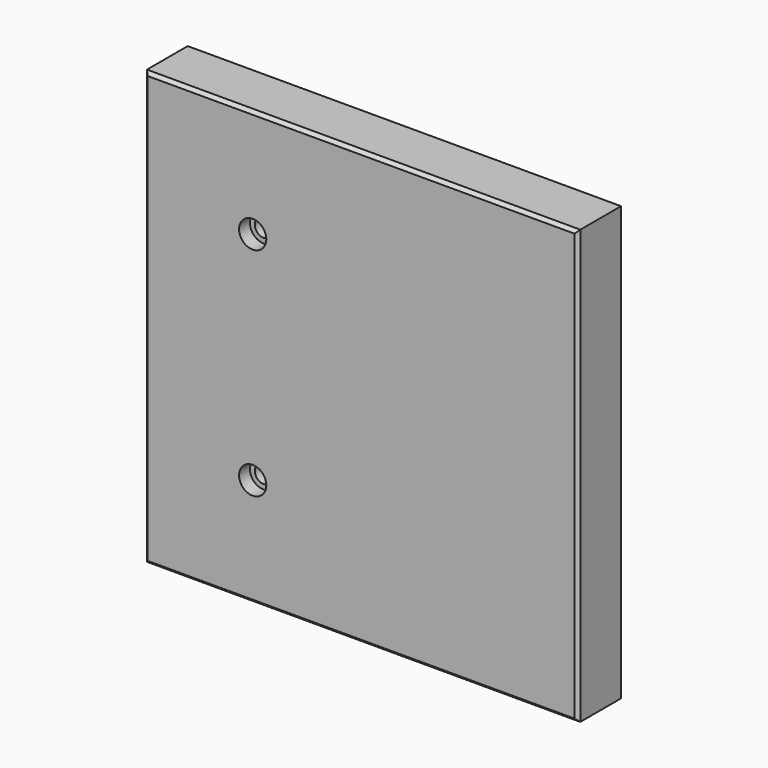
from build123d import *

# Parameters (mm, degrees)
F0_W     = 203.2
F0_H     = 203.2
F1_DEPTH = 12.7
F2_SIZE  = 1.524
F3_R     = 12.7
F4_DEPTH = 25.401
F5_R     = 12.7
F5_R_2   = 4.09575
F6_DEPTH = 12.7
F7_R     = 6.3754
F8_DEPTH = 6.35


# Not quite as in the source:
# - a pattern or mirror of a feature is missing from the dataset's text; its kind, count and spacing are read off the source's solid


with BuildPart() as f1:
    # F0 (on Front) → F1 (new body, symmetric)
    with BuildSketch(Plane.XZ):
        Rectangle(F0_W, F0_H)
    extrude(amount=F1_DEPTH, both=True)

    # F2
    f2_edges = [f1.edges().sort_by_distance(p)[0] for p in [
        (101.6, -12.7, 0),
        (0, -12.7, 101.6),
        (-101.6, -12.7, 0),
        (0, -12.7, -101.6),
    ]]
    chamfer(f2_edges, length=F2_SIZE)

    # F3 (on face) → F4 (cut, through all)
    with BuildSketch(Plane.XZ.offset(12.7)):
        with Locations((-50.8, -50.8)):
            Circle(F3_R)
    f4 = extrude(amount=-F4_DEPTH, mode=Mode.SUBTRACT)

    # F4_copies: F4 across plane
    add(f4.mirror(Plane.XY), mode=Mode.SUBTRACT)

    # F5 (on face) → F6 (join)
    with BuildSketch(Plane.XZ.offset(12.7)):
        with Locations((-50.8, 50.8)):
            Circle(F5_R)
        with Locations((-50.8, 50.8)):
            Circle(F5_R_2, mode=Mode.SUBTRACT)
        with Locations((-50.8, -50.8)):
            Circle(F5_R)
        with Locations((-50.8, -50.8)):
            Circle(F5_R_2, mode=Mode.SUBTRACT)
    extrude(amount=-F6_DEPTH)

    # F7 (on face) → F8 (cut)
    with BuildSketch(Plane.XZ.offset(12.7)):
        with Locations((-50.8, 50.8)):
            Circle(F7_R)
        with Locations((-50.8, -50.8)):
            Circle(F7_R)
    extrude(amount=-F8_DEPTH, mode=Mode.SUBTRACT)


solid = f1.part
